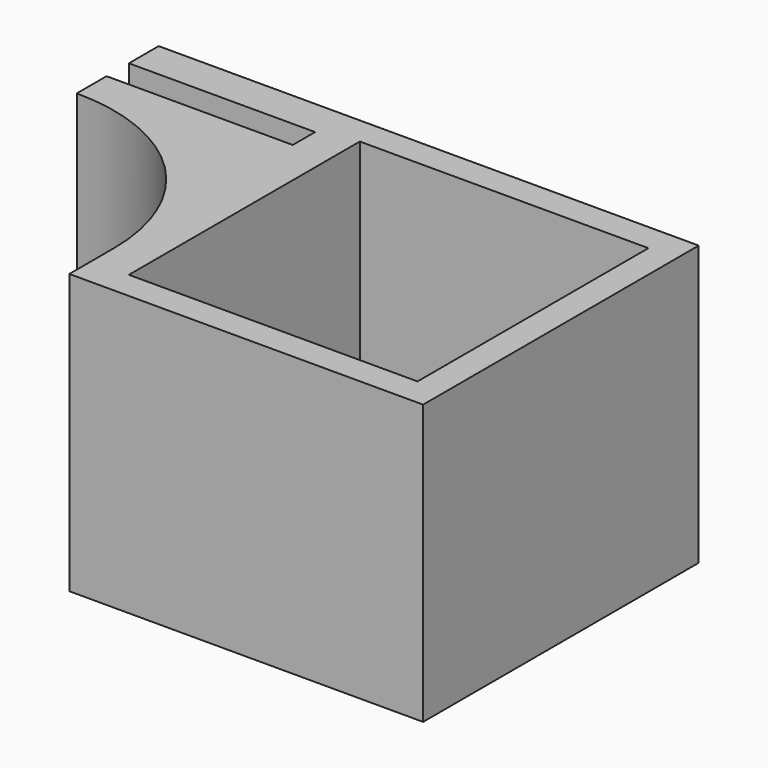
from build123d import *

# Parameters (mm, degrees)
F0_W     = 15.5
F0_H     = 15.5
F1_DEPTH = 7.5
F2_R     = 9.99999


# Not quite as in the source:
# - a fillet or chamfer is up to 0.001 mm smaller than in the source, because OpenCascade refuses the exact size
# - a feature names something its author has since deleted; it is built from what else it names


with BuildPart() as f1:
    # F0 (on Top) → F1 (new body, symmetric)
    with BuildSketch(Plane.XY):
        Polygon((-25.621605996, -0.5219928448), (-25.621605996, -7.0219928448), (-25.621605996, -13.5219928448), (-6.621605996, -13.5219928448), (-6.621605996, -8.299067306), (-6.621605996, 4.9780071552), (-35.621605996, 4.9780071552), (-35.621605996, 2.9780071552), (-25.621605996, 2.9780071552), (-25.621605996, 1.4780071552), (-35.621605996, 1.4780071552), (-35.621605996, -0.5219928448), align=None)
        with Locations((-15.871605996, -4.2719928448)):
            Rectangle(F0_W, F0_H, mode=Mode.SUBTRACT)
    extrude(amount=F1_DEPTH, both=True)

    # F2 (radius 10 in the source; OpenCascade refuses exactly that, so slightly less here)
    f2_edges = [f1.edges().sort_by_distance(p)[0] for p in [
        (-25.621606, -0.521993, 0),
    ]]
    fillet(f2_edges, radius=F2_R)


solid = f1.part
